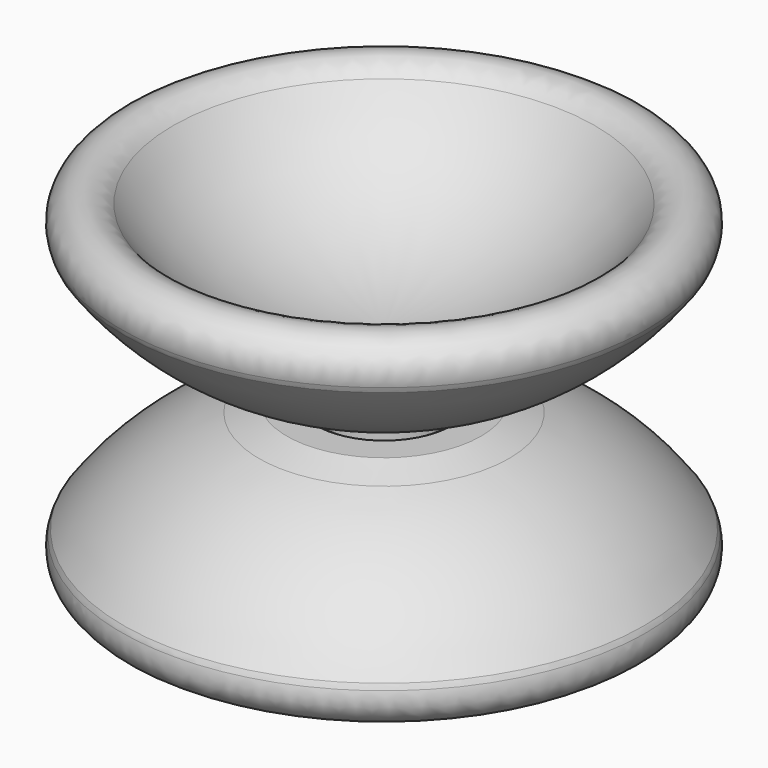
from build123d import *

# Parameters (mm, degrees)
F0_W            = 1.05
F0_H            = 3.6
F1_COPIES_COUNT = 9
F0_W_2          = 2
F3_R            = 26.492
F5_R            = 3


# Not quite as in the source:
# - a fillet or chamfer that OpenCascade refuses, or shapes differently, is made with other operations: its cross-section is extruded or revolved along the edge and cut away or added
# - a pattern or mirror of a feature is missing from the dataset's text; its kind, count and spacing are read off the source's solid


with BuildPart() as f1:
    # F0 (on Front) → F1 (revolve)
    with BuildSketch(Plane.XZ):
        with Locations((3.775, 20)):
            Rectangle(F0_W, F0_H)
    revolve(axis=Axis((3.25, 0, 20), (0, 0, -1)))


with BuildPart() as f1_copies_1:
    # F1_copies: instance of F1
    add(f1.part.rotate(Axis((0, 0, 0), (0, 0, 1)), 1 * 360 / F1_COPIES_COUNT))


with BuildPart() as f1_copies_2:
    # F1_copies: instance of F1
    add(f1.part.rotate(Axis((0, 0, 0), (0, 0, 1)), 2 * 360 / F1_COPIES_COUNT))


with BuildPart() as f1_copies_3:
    # F1_copies: instance of F1
    add(f1.part.rotate(Axis((0, 0, 0), (0, 0, 1)), 3 * 360 / F1_COPIES_COUNT))


with BuildPart() as f1_copies_4:
    # F1_copies: instance of F1
    add(f1.part.rotate(Axis((0, 0, 0), (0, 0, 1)), 4 * 360 / F1_COPIES_COUNT))


with BuildPart() as f1_copies_5:
    # F1_copies: instance of F1
    add(f1.part.rotate(Axis((0, 0, 0), (0, 0, 1)), 5 * 360 / F1_COPIES_COUNT))


with BuildPart() as f1_copies_6:
    # F1_copies: instance of F1
    add(f1.part.rotate(Axis((0, 0, 0), (0, 0, 1)), 6 * 360 / F1_COPIES_COUNT))


with BuildPart() as f1_copies_7:
    # F1_copies: instance of F1
    add(f1.part.rotate(Axis((0, 0, 0), (0, 0, 1)), 7 * 360 / F1_COPIES_COUNT))


with BuildPart() as f1_copies_8:
    # F1_copies: instance of F1
    add(f1.part.rotate(Axis((0, 0, 0), (0, 0, 1)), 8 * 360 / F1_COPIES_COUNT))


with BuildPart() as f2:
    # F0 (on Front) → F2 (revolve)
    with BuildSketch(Plane.XZ):
        with Locations((5.5, 20)):
            Rectangle(F0_W_2, F0_H)
    revolve(axis=Axis((0, 0, 15.4016362503), (0, 0, 1)))


with BuildPart() as f2b:
    # F0 (on Front) → F2, piece 2 (revolve)
    with BuildSketch(Plane.XZ):
        Polygon((2, 18), (2, 22), (7, 22), (7, 21.5), (10, 21.5), (23.831475452, 26.6078643763), (30, 40), (24, 40), (15, 25), (0, 25), (0, 15), (15, 15), (24, 0), (30, 0), (23.831475452, 13.3921356237), (10, 18.5), (7, 18.5), (7, 18), align=None)
    revolve(axis=Axis((0, 0, 15.4016362503), (0, 0, 1)))

    # F3
    f3_edges = [f2b.edges().sort_by_distance(p)[0] for p in [
        (-15, 0, 25),
        (-15, 0, 15),
    ]]
    fillet(f3_edges, radius=F3_R)

    # F4: fillet of radius 5 on 2 edges, made by hand

    # F4_s1 → F4_t2 (revolve, cut)
    with BuildSketch(Plane.XZ):
        with BuildLine():
            ThreePointArc((26.8665132304, 6.8029363371), (26.9327732416, 2.7696256765), (24, 0))
            Line((24, 0), (30, 0))
            Line((30, 0), (26.8665132304, 6.8029363371))
        make_face()
    revolve(axis=Axis((0, 0, 0), (0, 0, 1)), mode=Mode.SUBTRACT)

    # F4_s3 → F4_t4 (revolve, cut)
    with BuildSketch(Plane.XZ):
        with BuildLine():
            ThreePointArc((24, 40), (26.9327732416, 37.2303743235), (26.8665132304, 33.1970636629))
            Line((26.8665132304, 33.1970636629), (30, 40))
            Line((30, 40), (24, 40))
        make_face()
    revolve(axis=Axis((0, 0, 40), (0, 0, 1)), mode=Mode.SUBTRACT)

    # F5
    f5_edges = [f2b.edges().sort_by_distance(p)[0] for p in [
        (-24, 0, 40),
        (-24, 0, 0),
    ]]
    fillet(f5_edges, radius=F5_R)

    # F6: fillet of radius 30 on 2 edges, made by hand

    # F6_s1 → F6_t2 (revolve, cut)
    with BuildSketch(Plane.XZ):
        with BuildLine():
            ThreePointArc((26.8665132304, 33.1970636629), (20.679903748, 26.8416474974), (12.905362163, 22.5729293447))
            Line((12.905362163, 22.5729293447), (23.831475452, 26.6078643763))
            Line((23.831475452, 26.6078643763), (26.8665132304, 33.1970636629))
        make_face()
    revolve(axis=Axis((0, 0, 26.6078643763), (0, 0, 1)), mode=Mode.SUBTRACT)

    # F6_s3 → F6_t4 (revolve, cut)
    with BuildSketch(Plane.XZ):
        with BuildLine():
            ThreePointArc((12.905362163, 17.4270706553), (20.679903748, 13.1583525026), (26.8665132304, 6.8029363371))
            Line((26.8665132304, 6.8029363371), (23.831475452, 13.3921356237))
            Line((23.831475452, 13.3921356237), (12.905362163, 17.4270706553))
        make_face()
    revolve(axis=Axis((0, 0, 13.3921356237), (0, 0, 1)), mode=Mode.SUBTRACT)


solid = Compound([f1.part, f1_copies_1.part, f1_copies_2.part, f1_copies_3.part, f1_copies_4.part, f1_copies_5.part, f1_copies_6.part, f1_copies_7.part, f1_copies_8.part, f2.part, f2b.part])
